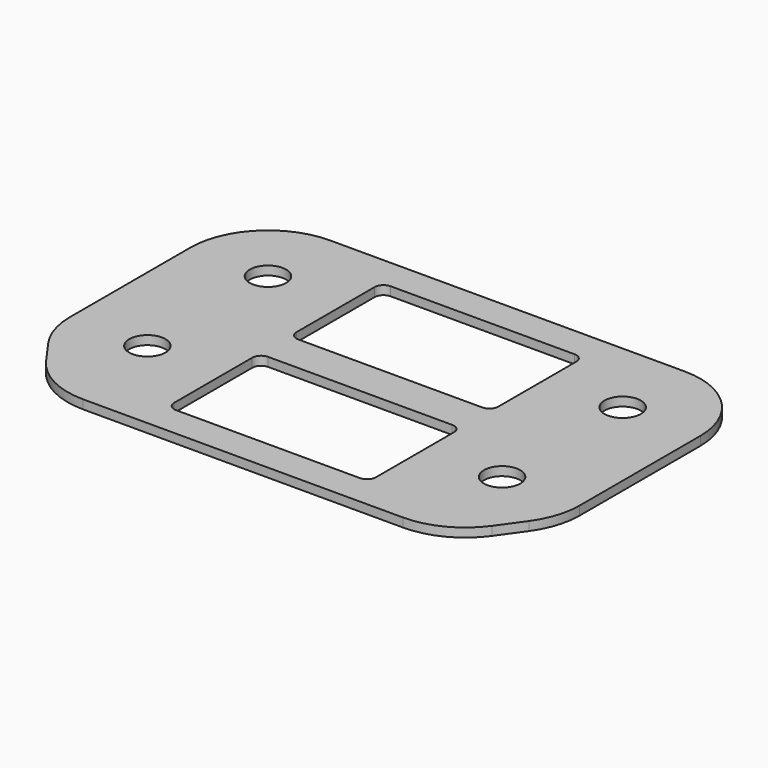
from build123d import *

# Parameters (mm, degrees)
F0_R     = 12.5
F0_W     = 22.75
F0_H     = 26
F1_DEPTH = 2
F2_DEPTH = 25
F3_R     = 2
F4_D     = 8.2


# Not quite as in the source:
# - a feature names something its author has since deleted; it is built from what else it names


with BuildPart() as f1:
    # F0 (on Top) → F1 (new body)
    with BuildSketch(Plane.XY):
        with BuildLine():
            Line((-22.75, 1.5), (-22.75, 27.5))
            Line((-22.75, 27.5), (0, 27.5))
            Line((0, 27.5), (0, 34.5))
            Line((0, 34.5), (-40, 34.5))
            ThreePointArc((-40, 34.5), (-52.3743686708, 29.3743686708), (-57.5, 17))
            Line((-57.5, 17), (-57.5, -17))
            ThreePointArc((-57.5, -17), (-56.6642107828, -22.3436016868), (-54.2366766871, -27.1767891256))
            Line((-54.2366766871, -27.1767891256), (-50.3051172775, -32.6767891256))
            ThreePointArc((-50.3051172775, -32.6767891256), (-44.0733200493, -38.0618734363), (-36.0684405904, -40))
            Line((-36.0684405904, -40), (0, -40))
            Line((0, -40), (0, -33))
            Line((0, -33), (-22.75, -33))
            Line((-22.75, -33), (-22.75, -7))
            Line((-22.75, -7), (0, -7))
            Line((0, -7), (0, 1.5))
            Line((0, 1.5), (-22.75, 1.5))
        make_face()
        with Locations((-40, -17)):
            Circle(F0_R, mode=Mode.SUBTRACT)
        with Locations((-40, 17)):
            Circle(F0_R, mode=Mode.SUBTRACT)
        with Locations((-11.375, 14.5)):
            Rectangle(F0_W, F0_H)
        with Locations((-11.375, -20)):
            Rectangle(F0_W, F0_H)
        with Locations((-40, 17)):
            Circle(F0_R)
        with Locations((-40, -17)):
            Circle(F0_R)
    extrude(amount=F1_DEPTH)

    # F0 (on Top) → F2 (cut)
    with BuildSketch(Plane.XY):
        with Locations((-11.375, 14.5)):
            Rectangle(F0_W, F0_H)
        with Locations((-11.375, -20)):
            Rectangle(F0_W, F0_H)
    extrude(amount=F2_DEPTH, mode=Mode.SUBTRACT)

    # F3
    f3_edges = [f1.edges().sort_by_distance(p)[0] for p in [
        (-22.75, 1.5, 1),
        (-22.75, 27.5, 1),
        (-22.75, -7, 1),
        (-22.75, -33, 1),
    ]]
    fillet(f3_edges, radius=F3_R)

    # F4 (through all)
    with Locations(Plane(origin=(0, 0, 0), x_dir=(1, 0, 0), z_dir=(0, 0, -1))):
        with Locations((-40, -17), (-40, 17)):
            Hole(F4_D / 2)

    # F5: F1 across plane


with BuildPart() as f1_1:
    add(f1.part)
    add(f1.part.mirror(Plane.YZ))


solid = f1_1.part
